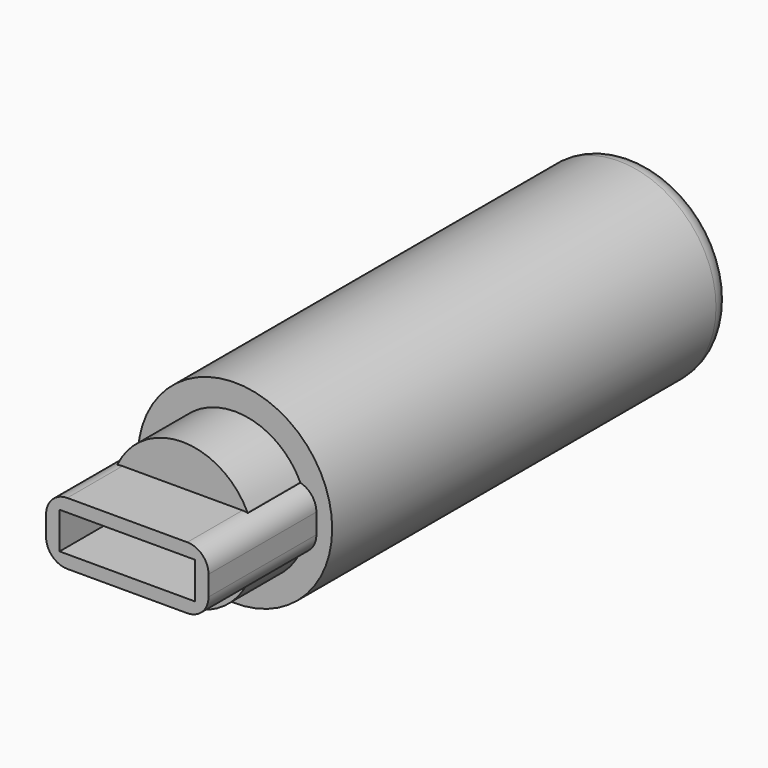
from build123d import *

# Parameters (mm, degrees)
F0_R         = 23.2504682004
F0_R_2       = 17.1266274378
F1_DEPTH     = 59.944
F2_R         = 5.08
F4_W         = 32.4101708829
F4_H         = 8.7824892253
F5_DEPTH     = 32.258
F6_W         = 31.7728198101
F6_H         = 11.3427176839
F6_W_2       = 31.0806287388
F6_H_2       = 14.8886315292
F7_DEPTH     = 16.51
F8_T4_DEPTH  = 57.658
F8_T9_DEPTH  = 44.958
F8_S10_R     = 17.2448690912
F8_T11_DEPTH = 24
F8_T15_DEPTH = 44.958
F8_S16_R     = 17.2448690912
F8_T17_DEPTH = 24
F8_T21_DEPTH = 57.658
F8_T26_DEPTH = 44.958
F8_S27_R     = 17.2448690912
F8_T28_DEPTH = 24
F8_T32_DEPTH = 57.658
F8_T37_DEPTH = 44.958
F8_S38_R     = 17.2448690912
F8_T39_DEPTH = 24
F8_T43_DEPTH = 57.658


# Not quite as in the source:
# - a fillet or chamfer that OpenCascade refuses, or shapes differently, is made with other operations: its cross-section is extruded or revolved along the edge and cut away or added


with BuildPart() as f1:
    # F0 (on Front) → F1 (new body, symmetric)
    with BuildSketch(Plane.XZ):
        with Locations((-0.0308285998, 0.0824332965)):
            Circle(F0_R)
        Circle(F0_R_2, mode=Mode.SUBTRACT)
    extrude(amount=F1_DEPTH, both=True)

    # F2
    f2_edges = [f1.edges().sort_by_distance(p)[0] for p in [
        (-23.281297, 59.944, 0.082433),
    ]]
    fillet(f2_edges, radius=F2_R)

    # F4 (on face) → F5 (join)
    with BuildSketch(Plane.XZ.offset(59.944)):
        Polygon((-15.5403143694, 7.475569495), (-19.4364797935, 7.475569495), (-19.4364797935, -7.475569495), (-15.5403143694, -7.475569495), (15.5403143694, -7.475569495), (19.4364797935, -7.475569495), (19.4364797935, 7.475569495), (15.5403143694, 7.475569495), align=None)
        Rectangle(F4_W, F4_H, mode=Mode.SUBTRACT)
        with BuildLine():
            ThreePointArc((15.5403143694, 7.475569495), (0, 17.2448690912), (-15.5403143694, 7.475569495))
            Line((-15.5403143694, 7.475569495), (15.5403143694, 7.475569495))
        make_face()
        with BuildLine():
            Line((15.5403143694, -7.475569495), (-15.5403143694, -7.475569495))
            ThreePointArc((-15.5403143694, -7.475569495), (0, -17.2448690912), (15.5403143694, -7.475569495))
        make_face()
    extrude(amount=F5_DEPTH)

    # F6 (on face) → F7 (cut)
    with BuildSketch(Plane.XZ.offset(92.202)):
        with Locations((0.3460955357, 13.1469283369)):
            Rectangle(F6_W, F6_H)
        with Locations((0, -14.9198852596)):
            Rectangle(F6_W_2, F6_H_2)
    extrude(amount=-F7_DEPTH, mode=Mode.SUBTRACT)

    # F8: fillet of radius 5.08 on 4 edges, made by hand


with BuildPart() as f8_tool2:
    # F8_s3 → F8_t4 (new body)
    with BuildSketch(Plane.XZ.offset(47.244)):
        with BuildLine():
            ThreePointArc((-14.3564797935, -7.475569495), (-17.9485822419, -5.9876719434), (-19.4364797935, -2.395569495))
            Line((-19.4364797935, -2.395569495), (-19.4364797935, -7.475569495))
            Line((-19.4364797935, -7.475569495), (-14.3564797935, -7.475569495))
        make_face()
    extrude(amount=F8_T4_DEPTH)

    split(bisect_by=Plane.XZ.offset(75.692), keep=Keep.TOP)


with BuildPart() as f1_1:
    add(f1.part)

    # F8_t1: cut F8_tool2
    add(f8_tool2.part, mode=Mode.SUBTRACT)


with BuildPart() as f8_tool7:
    # F8_s8 → F8_t9 (new body)
    with BuildSketch(Plane.XZ.offset(59.944)):
        with BuildLine():
            ThreePointArc((-14.3564797935, -7.475569495), (-17.9485822419, -5.9876719434), (-19.4364797935, -2.395569495))
            Line((-19.4364797935, -2.395569495), (-19.4364797935, -7.475569495))
            Line((-19.4364797935, -7.475569495), (-14.3564797935, -7.475569495))
        make_face()
    extrude(amount=F8_T9_DEPTH)

    # F8_s10 → F8_t11 (cut, symmetric)
    with BuildSketch(Plane.XZ.offset(82.4)):
        Circle(F8_S10_R)
    extrude(amount=F8_T11_DEPTH, both=True, mode=Mode.SUBTRACT)


with BuildPart() as f1_2:
    add(f1_1.part)

    # F8_t6: cut F8_tool7
    add(f8_tool7.part, mode=Mode.SUBTRACT)


with BuildPart() as f8_tool13:
    # F8_s14 → F8_t15 (new body)
    with BuildSketch(Plane.XZ.offset(59.944)):
        with BuildLine():
            ThreePointArc((19.4364797935, -2.395569495), (17.9485822419, -5.9876719434), (14.3564797935, -7.475569495))
            Line((14.3564797935, -7.475569495), (19.4364797935, -7.475569495))
            Line((19.4364797935, -7.475569495), (19.4364797935, -2.395569495))
        make_face()
    extrude(amount=F8_T15_DEPTH)

    # F8_s16 → F8_t17 (cut, symmetric)
    with BuildSketch(Plane.XZ.offset(82.4)):
        Circle(F8_S16_R)
    extrude(amount=F8_T17_DEPTH, both=True, mode=Mode.SUBTRACT)


with BuildPart() as f1_3:
    add(f1_2.part)

    # F8_t12: cut F8_tool13
    add(f8_tool13.part, mode=Mode.SUBTRACT)


with BuildPart() as f8_tool19:
    # F8_s20 → F8_t21 (new body)
    with BuildSketch(Plane.XZ.offset(47.244)):
        with BuildLine():
            ThreePointArc((19.4364797935, -2.395569495), (17.9485822419, -5.9876719434), (14.3564797935, -7.475569495))
            Line((14.3564797935, -7.475569495), (19.4364797935, -7.475569495))
            Line((19.4364797935, -7.475569495), (19.4364797935, -2.395569495))
        make_face()
    extrude(amount=F8_T21_DEPTH)

    split(bisect_by=Plane.XZ.offset(75.692), keep=Keep.TOP)


with BuildPart() as f1_4:
    add(f1_3.part)

    # F8_t18: cut F8_tool19
    add(f8_tool19.part, mode=Mode.SUBTRACT)


with BuildPart() as f8_tool24:
    # F8_s25 → F8_t26 (new body)
    with BuildSketch(Plane.XZ.offset(59.944)):
        with BuildLine():
            ThreePointArc((19.4364797935, 2.395569495), (17.9485822419, 5.9876719434), (14.3564797935, 7.475569495))
            Line((14.3564797935, 7.475569495), (19.4364797935, 7.475569495))
            Line((19.4364797935, 7.475569495), (19.4364797935, 2.395569495))
        make_face()
    extrude(amount=F8_T26_DEPTH)

    # F8_s27 → F8_t28 (cut, symmetric)
    with BuildSketch(Plane.XZ.offset(82.4)):
        Circle(F8_S27_R)
    extrude(amount=F8_T28_DEPTH, both=True, mode=Mode.SUBTRACT)


with BuildPart() as f1_5:
    add(f1_4.part)

    # F8_t23: cut F8_tool24
    add(f8_tool24.part, mode=Mode.SUBTRACT)


with BuildPart() as f8_tool30:
    # F8_s31 → F8_t32 (new body)
    with BuildSketch(Plane.XZ.offset(47.244)):
        with BuildLine():
            ThreePointArc((19.4364797935, 2.395569495), (17.9485822419, 5.9876719434), (14.3564797935, 7.475569495))
            Line((14.3564797935, 7.475569495), (19.4364797935, 7.475569495))
            Line((19.4364797935, 7.475569495), (19.4364797935, 2.395569495))
        make_face()
    extrude(amount=F8_T32_DEPTH)

    split(bisect_by=Plane.XZ.offset(75.692), keep=Keep.TOP)


with BuildPart() as f1_6:
    add(f1_5.part)

    # F8_t29: cut F8_tool30
    add(f8_tool30.part, mode=Mode.SUBTRACT)


with BuildPart() as f8_tool35:
    # F8_s36 → F8_t37 (new body)
    with BuildSketch(Plane.XZ.offset(59.944)):
        with BuildLine():
            ThreePointArc((-19.4364797935, 2.395569495), (-17.9485822419, 5.9876719434), (-14.3564797935, 7.475569495))
            Line((-14.3564797935, 7.475569495), (-19.4364797935, 7.475569495))
            Line((-19.4364797935, 7.475569495), (-19.4364797935, 2.395569495))
        make_face()
    extrude(amount=F8_T37_DEPTH)

    # F8_s38 → F8_t39 (cut, symmetric)
    with BuildSketch(Plane.XZ.offset(82.4)):
        Circle(F8_S38_R)
    extrude(amount=F8_T39_DEPTH, both=True, mode=Mode.SUBTRACT)


with BuildPart() as f1_7:
    add(f1_6.part)

    # F8_t34: cut F8_tool35
    add(f8_tool35.part, mode=Mode.SUBTRACT)


with BuildPart() as f8_tool41:
    # F8_s42 → F8_t43 (new body)
    with BuildSketch(Plane.XZ.offset(47.244)):
        with BuildLine():
            ThreePointArc((-19.4364797935, 2.395569495), (-17.9485822419, 5.9876719434), (-14.3564797935, 7.475569495))
            Line((-14.3564797935, 7.475569495), (-19.4364797935, 7.475569495))
            Line((-19.4364797935, 7.475569495), (-19.4364797935, 2.395569495))
        make_face()
    extrude(amount=F8_T43_DEPTH)

    split(bisect_by=Plane.XZ.offset(75.692), keep=Keep.TOP)


with BuildPart() as f1_8:
    add(f1_7.part)

    # F8_t40: cut F8_tool41
    add(f8_tool41.part, mode=Mode.SUBTRACT)


solid = f1_8.part
